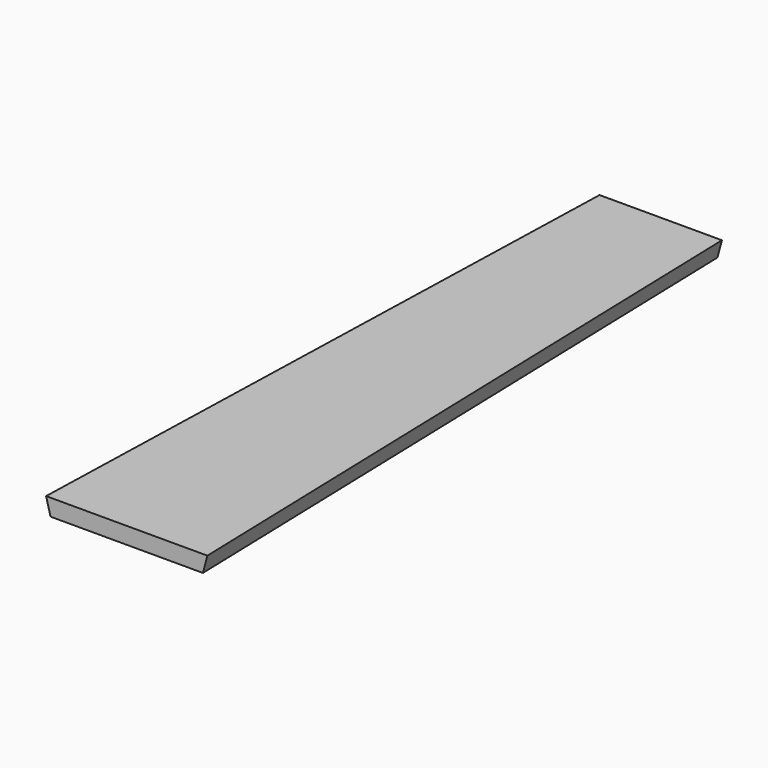
from build123d import *

# Parameters (mm, degrees)
F1_DEPTH = 19.05


with BuildPart() as f1:
    # F0 (on Top) → F1 (new body)
    with BuildSketch(Plane.XY):
        Polygon((22.2249564553, 762), (0, 0), (184.15, 0), (161.9249564553, 762), align=None)
    extrude(amount=F1_DEPTH)

    # F2 (on face) → F4 section 0
    with BuildSketch(Plane(origin=(0, 762, 0), x_dir=(-1, 0, 0), z_dir=(0, 1, 0))):
        Polygon((-156.8205243395, 0), (-161.9249564553, 19.05), (-161.9249564553, 0), align=None)
    # F3 (on face) → F4 section 1
    with BuildSketch(Plane.XZ):
        Polygon((184.15, 0), (184.15, 19.05), (179.0455678842, 0), align=None)
    loft(mode=Mode.SUBTRACT)

    # F5 (on face) → F7 section 0
    with BuildSketch(Plane.XZ):
        Polygon((0, 19.05), (0, 0), (5.1044321158, 0), align=None)
    # F6 (on face) → F7 section 1
    with BuildSketch(Plane(origin=(0, 762, 0), x_dir=(-1, 0, 0), z_dir=(0, 1, 0))):
        Polygon((-22.2249564553, 0), (-22.2249564553, 19.05), (-27.3293885711, 0), align=None)
    loft(mode=Mode.SUBTRACT)


solid = f1.part
